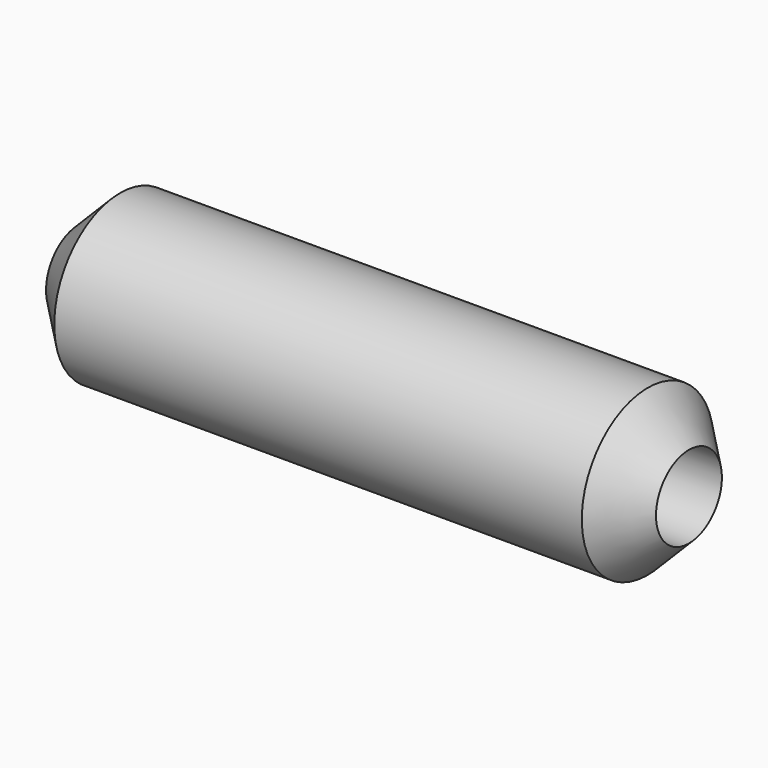
from build123d import *

# Parameters (mm, degrees)
F0_R     = 6.35
F0_R_2   = 3.175
F1_DEPTH = 50.8


# Not quite as in the source:
# - a fillet or chamfer that OpenCascade refuses, or shapes differently, is made with other operations: its cross-section is extruded or revolved along the edge and cut away or added


with BuildPart() as f1:
    # F0 (on Right) → F1 (new body)
    with BuildSketch(Plane.YZ):
        Circle(F0_R)
        Circle(F0_R_2, mode=Mode.SUBTRACT)
    extrude(amount=F1_DEPTH)

    # F2: chamfer of 5.08 on 3 edges, made by hand

    # F2_s1 → F2_t2 (revolve, cut)
    with BuildSketch(Plane.XY):
        Polygon((45.72, 6.35), (50.8, 1.27), (50.8, 6.35), align=None)
    revolve(axis=Axis((50.8, 0, 0), (1, 0, 0)), mode=Mode.SUBTRACT)

    # F2_s3 → F2_t4 (revolve, cut)
    with BuildSketch(Plane.XY):
        Polygon((5.08, 6.35), (0, 1.27), (0, 6.35), align=None)
    revolve(axis=Axis((0, 0, 0), (1, 0, 0)), mode=Mode.SUBTRACT)


solid = f1.part
